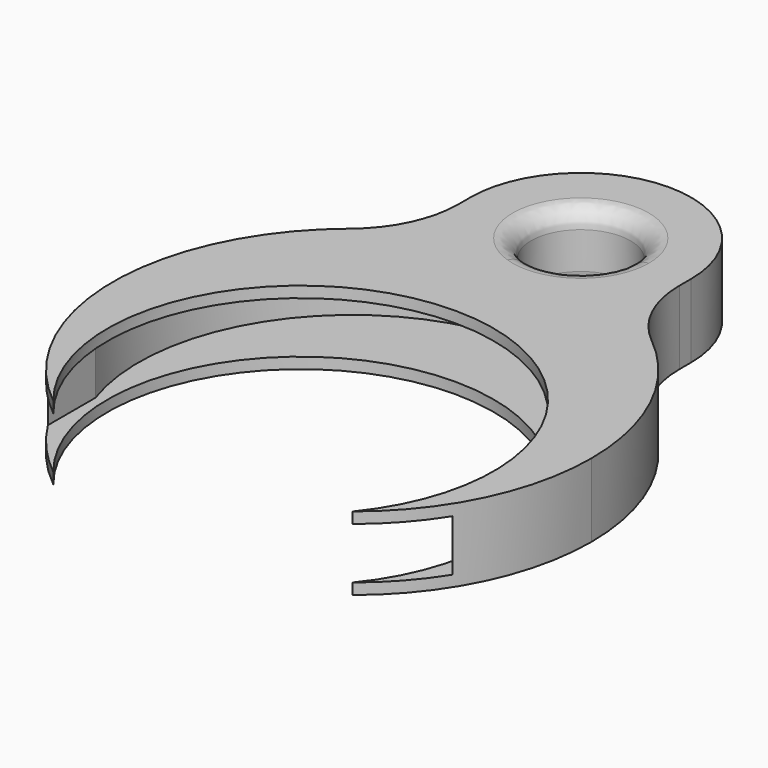
from build123d import *

# Parameters (mm, degrees)
F1_DEPTH = 2
F2_R     = 5.99999
F3_R     = 1
F4_R     = 10.5
F5_DEPTH = 4.001
F7_DEPTH = 1.4


# Not quite as in the source:
# - a fillet or chamfer is up to 0.001 mm smaller than in the source, because OpenCascade refuses the exact size


with BuildPart() as f1:
    # F0 (on Top) → F1 (new body, symmetric)
    with BuildSketch(Plane.XY):
        with BuildLine():
            ThreePointArc((-6, 11.5325625947), (-6.7453687816, -11.1130553854), (13, 0))
            ThreePointArc((13, 0), (11.1130553854, 6.7453687816), (6, 11.5325625947))
            Line((6, 11.5325625947), (-6, 11.5325625947))
        make_face()
        with BuildLine():
            Line((-6, 11.5325625947), (6, 11.5325625947))
            ThreePointArc((6, 11.5325625947), (3.5026447844, 12.5192443667), (0.8558504936, 12.9717970973))
            ThreePointArc((0.8558504936, 12.9717970973), (0, 12.8325625947), (-0.8558504936, 12.9717970973))
            ThreePointArc((-0.8558504936, 12.9717970973), (-3.5026447844, 12.5192443667), (-6, 11.5325625947))
        make_face()
        with BuildLine():
            ThreePointArc((0.8558504936, 12.9717970973), (3.5026447844, 12.5192443667), (6, 11.5325625947))
            Line((6, 11.5325625947), (6, 21.5325625947))
            Line((6, 21.5325625947), (-6, 21.5325625947))
            Line((-6, 21.5325625947), (-6, 11.5325625947))
            ThreePointArc((-6, 11.5325625947), (-3.5026447844, 12.5192443667), (-0.8558504936, 12.9717970973))
            ThreePointArc((-0.8558504936, 12.9717970973), (-1.5778472149, 17.7235436914), (2.7, 15.5325625947))
            ThreePointArc((2.7, 15.5325625947), (2.1909810967, 13.9547153797), (0.8558504936, 12.9717970973))
        make_face()
    extrude(amount=F1_DEPTH, both=True)

    # F2 (radius 6 in the source; OpenCascade refuses exactly that, so slightly less here)
    f2_edges = [f1.edges().sort_by_distance(p)[0] for p in [
        (-6, 21.532563, 0),
        (6, 21.532563, 0),
        (6, 11.532563, 0),
        (-6, 11.532563, 0),
    ]]
    fillet(f2_edges, radius=F2_R)

    # F3
    f3_edges = [f1.edges().sort_by_distance(p)[0] for p in [
        (0.85585, 18.093328, 2),
        (0.85585, 18.093328, -2),
    ]]
    fillet(f3_edges, radius=F3_R)

    # F4 (on face) → F5 (cut, through all)
    with BuildSketch(Plane.XY.offset(2)):
        with Locations((0, -3.5)):
            Circle(F4_R)
    extrude(amount=-F5_DEPTH, mode=Mode.SUBTRACT)

    # F6 (on Top) → F7 (cut, symmetric)
    with BuildSketch(Plane.XY):
        with BuildLine():
            ThreePointArc((11, -3.6981110043), (11.452751307, -1.8736361707), (11.605, 0))
            ThreePointArc((11.605, 0), (-1.8736361707, 11.452751307), (-11, -3.6981110043))
            Line((-11, -3.6981110043), (11, -3.6981110043))
        make_face()
        with BuildLine():
            Line((11, -3.6981110043), (-11, -3.6981110043))
            ThreePointArc((-11, -3.6981110043), (0, -11.605), (11, -3.6981110043))
        make_face()
        with BuildLine():
            ThreePointArc((11, -3.6981110043), (0, -11.605), (-11, -3.6981110043))
            Line((-11, -3.6981110043), (-11, -14.1476519146))
            Line((-11, -14.1476519146), (11, -14.1476519146))
            Line((11, -14.1476519146), (11, -3.6981110043))
        make_face()
    extrude(amount=F7_DEPTH, both=True, mode=Mode.SUBTRACT)


solid = f1.part
